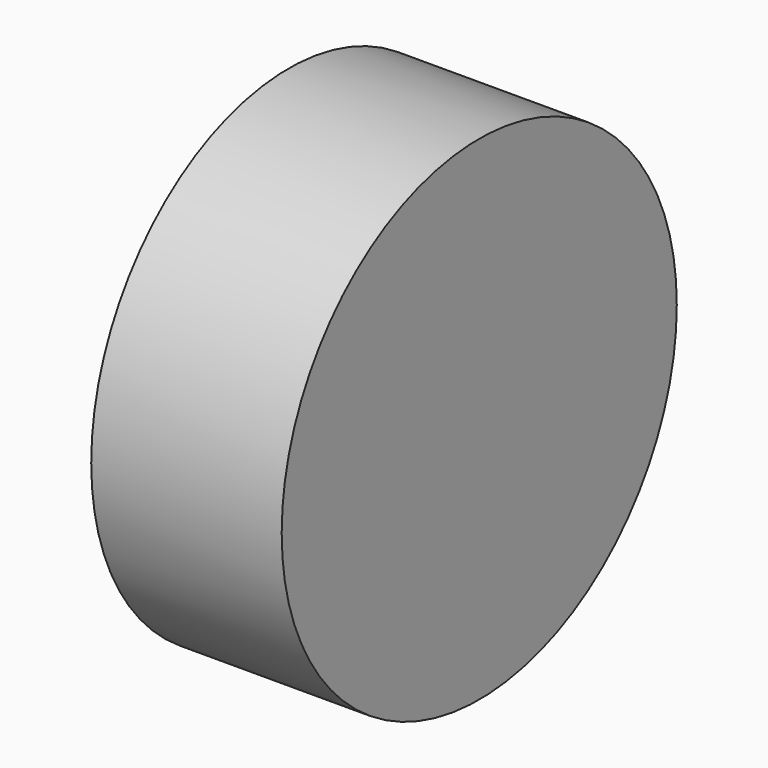
from build123d import *

# Parameters (mm, degrees)
F0_W = 67.9279565811
F0_H = 88.0647003651


# Not quite as in the source:
# - a feature of the source that left no trace in its solid (it failed there, or was rolled back) is left out


with BuildPart() as f1:
    # F0 (on Top) → F1 (revolve)
    with BuildSketch(Plane.XY):
        Rectangle(F0_W, F0_H)
    revolve(axis=Axis((0, -44.0323501825, 0), (-1, 0, 0)))


solid = f1.part
